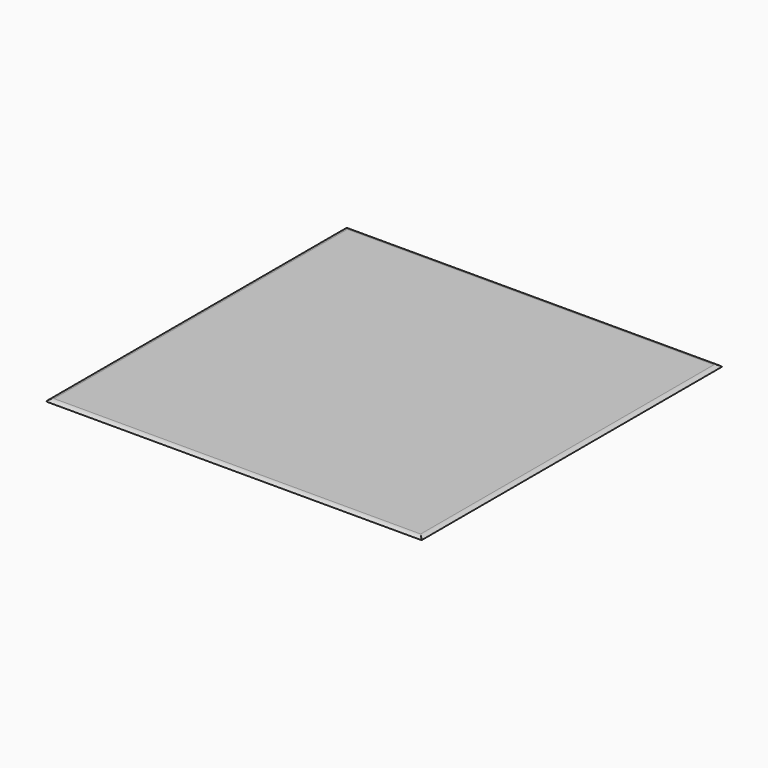
from build123d import *

# Parameters (mm, degrees)
F0_W        = 340
F0_H        = 340
F1_DEPTH    = 2
F2_T1_DEPTH = 360
F2_T3_DEPTH = 360


# Not quite as in the source:
# - a fillet or chamfer that OpenCascade refuses, or shapes differently, is made with other operations: its cross-section is extruded or revolved along the edge and cut away or added


with BuildPart() as f1:
    # F0 (on Top) → F1 (new body)
    with BuildSketch(Plane.XY):
        Rectangle(F0_W, F0_H)
    extrude(amount=F1_DEPTH)

    # F2: fillet of radius 5 on 4 edges, made by hand

    # F2_s2 → F2_t1 (cut)
    with BuildSketch(Plane.XZ.offset(-180)):
        with BuildLine():
            ThreePointArc((170, 0), (168.2360679775, 1.472135955), (166, 2))
            Line((166, 2), (170, 2))
            Line((170, 2), (170, 0))
        make_face()
        with BuildLine():
            ThreePointArc((-170, 0), (-168.2360679775, 1.472135955), (-166, 2))
            Line((-166, 2), (-170, 2))
            Line((-170, 2), (-170, 0))
        make_face()
    extrude(amount=F2_T1_DEPTH, mode=Mode.SUBTRACT)

    # F2_s4 → F2_t3 (cut)
    with BuildSketch(Plane.YZ.offset(-180)):
        with BuildLine():
            ThreePointArc((-170, 0), (-168.2360679775, 1.472135955), (-166, 2))
            Line((-166, 2), (-170, 2))
            Line((-170, 2), (-170, 0))
        make_face()
        with BuildLine():
            ThreePointArc((170, 0), (168.2360679775, 1.472135955), (166, 2))
            Line((166, 2), (170, 2))
            Line((170, 2), (170, 0))
        make_face()
    extrude(amount=F2_T3_DEPTH, mode=Mode.SUBTRACT)


solid = f1.part
